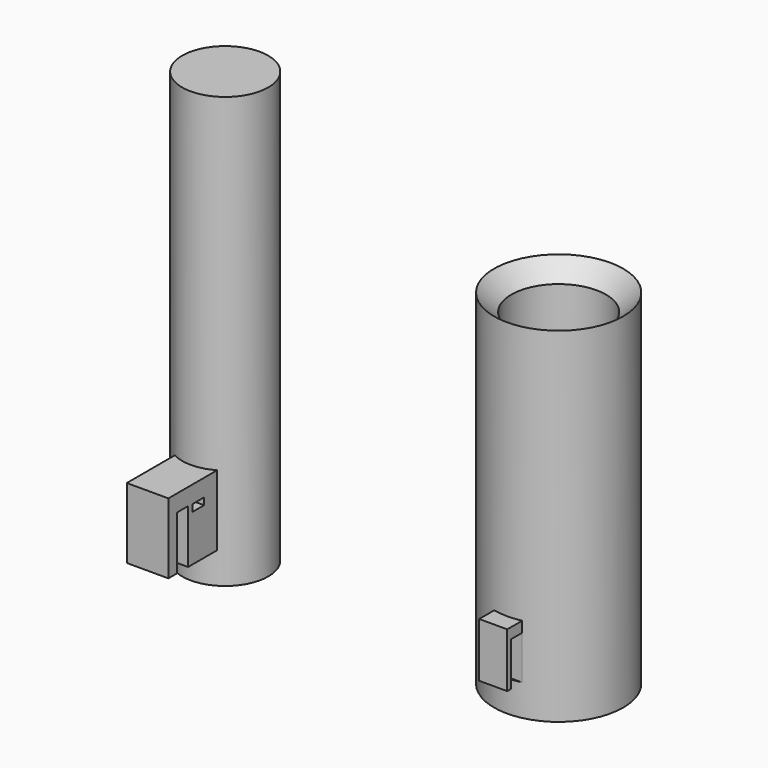
from build123d import *

# Parameters (mm, degrees)
F0_R      = 7.5
F1_DEPTH  = 40
F0_R_2    = 5
F2_DEPTH  = 50
F3_T      = -2
F5_W      = 4.8330873251
F5_H      = 8.1790685654
F6_DEPTH  = 3.9
F5_W_2    = 3.2551530749
F5_H_2    = 6.3201887533
F7_DEPTH  = 2
F8_W      = 1.0505022947
F8_H      = 0.8033253253
F8_W_2    = 0.6179423071
F9_DEPTH  = 4.8330873251
F10_W     = 1.6568034714
F10_H     = 5.0862235948
F11_DEPTH = 3.2551530749
F12_SIZE  = 1.99999
F13_W     = 1.6043800861
F13_H     = 6.2287077308
F14_DEPTH = 4.8330873251


# Not quite as in the source:
# - a fillet or chamfer is up to 0.001 mm smaller than in the source, because OpenCascade refuses the exact size
# - a feature names something its author has since deleted; it is built from what else it names


with BuildPart() as f1:
    # F0 (on Top) → F1 (new body)
    with BuildSketch(Plane.XY):
        Circle(F0_R)
    extrude(amount=F1_DEPTH)

    # F3
    f3_openings = [f1.faces().sort_by_distance(p)[0] for p in [
        (0, 0, 40),
    ]]
    offset(amount=F3_T, openings=f3_openings)

    # F5 (on offset) → F7 (join, symmetric)
    with BuildSketch(Plane.XZ.offset(7.5)):
        with Locations((0, 6.7948191427)):
            Rectangle(F5_W_2, F5_H_2)
    extrude(amount=F7_DEPTH, both=True)

    # F10 (on face) → F11 (cut, through all)
    with BuildSketch(Plane(origin=(-1.6275765374, 0, 0), x_dir=(0, -1, 0), z_dir=(-1, 0, 0))):
        with Locations((8.1496717495, 6.1778365634)):
            Rectangle(F10_W, F10_H)
    extrude(amount=-F11_DEPTH, mode=Mode.SUBTRACT)

    # F12 (size 2 in the source; OpenCascade refuses exactly that, so slightly less here)
    f12_edges = [f1.edges().sort_by_distance(p)[0] for p in [
        (-5.5, 0, 40),
    ]]
    chamfer(f12_edges, length=F12_SIZE)


with BuildPart() as f2:
    # F0 (on Top) → F2 (new body)
    with BuildSketch(Plane.XY):
        with Locations((-38.7259498239, 0)):
            Circle(F0_R_2)
    extrude(amount=F2_DEPTH)

    # F5 (on offset) → F6 (join, symmetric)
    with BuildSketch(Plane.XZ.offset(7.5)):
        with Locations((-38.6192724109, 7.7242590487)):
            Rectangle(F5_W, F5_H)
    extrude(amount=F6_DEPTH, both=True)

    # F8 (on face) → F9 (cut, through all)
    with BuildSketch(Plane(origin=(-41.0358160734, 0, 0), x_dir=(0, -1, 0), z_dir=(-1, 0, 0))):
        with Locations((7.3549995432, 9.4093019143)):
            Rectangle(F8_W, F8_H)
        with Locations((6.5207772423, 9.4093019143)):
            Rectangle(F8_W_2, F8_H)
    extrude(amount=-F9_DEPTH, mode=Mode.SUBTRACT)

    # F13 (on face) → F14 (cut, through all)
    with BuildSketch(Plane(origin=(-41.0358160734, 0, 0), x_dir=(0, -1, 0), z_dir=(-1, 0, 0))):
        with Locations((9.3433512375, 6.7490786314)):
            Rectangle(F13_W, F13_H)
    extrude(amount=-F14_DEPTH, mode=Mode.SUBTRACT)


solid = Compound([f1.part, f2.part])
